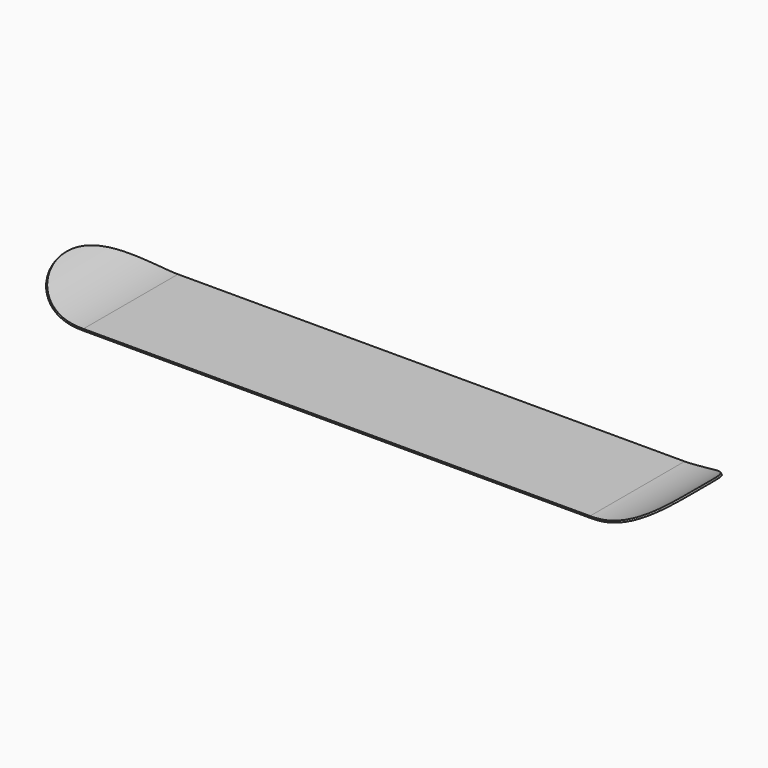
from build123d import *

# Parameters (mm, degrees)
F1_DEPTH    = 175
F2_T1_DEPTH = 875


# Not quite as in the source:
# - a fillet or chamfer that OpenCascade refuses, or shapes differently, is made with other operations: its cross-section is extruded or revolved along the edge and cut away or added


with BuildPart() as f1:
    # F0 (on Front) → F1 (new body, symmetric)
    with BuildSketch(Plane.XZ):
        with BuildLine():
            Line((-750, 0), (0, 0))
            Line((0, 0), (0, 5))
            Line((0, 5), (-750, 5))
            ThreePointArc((-750, 5), (-850.8959422811, 22.7906768682), (-939.6223448575, 74.0168892799))
            Line((-939.6223448575, 74.0168892799), (-942.836282906, 70.1866670643))
            ThreePointArc((-942.836282906, 70.1866670643), (-852.6060429977, 18.0922137642), (-750, 0))
        make_face()
    extrude(amount=F1_DEPTH, both=True)

    # F2: fillet of radius 174 on 2 edges, made by hand

    # F2_s2 → F2_t1 (cut)
    with BuildSketch(Plane(origin=(-72.170505067, 0, -86.0094586929), x_dir=(0, 1, 0), z_dir=(-0.6427876097, 0, -0.7660444431))):
        with BuildLine():
            ThreePointArc((-1, -767.3696152452), (-124.0365799265, -716.4061951717), (-175, -593.3696152452))
            Line((-175, -593.3696152452), (-175, -767.3696152452))
            Line((-175, -767.3696152452), (-1, -767.3696152452))
        make_face()
        with BuildLine():
            ThreePointArc((1, -767.3696152452), (124.0365799265, -716.4061951717), (175, -593.3696152452))
            Line((175, -593.3696152452), (175, -767.3696152452))
            Line((175, -767.3696152452), (1, -767.3696152452))
        make_face()
    extrude(amount=F2_T1_DEPTH, mode=Mode.SUBTRACT)

    # F3: F1 across plane


with BuildPart() as f1_1:
    add(f1.part)
    add(f1.part.mirror(Plane.YZ))


solid = f1_1.part
